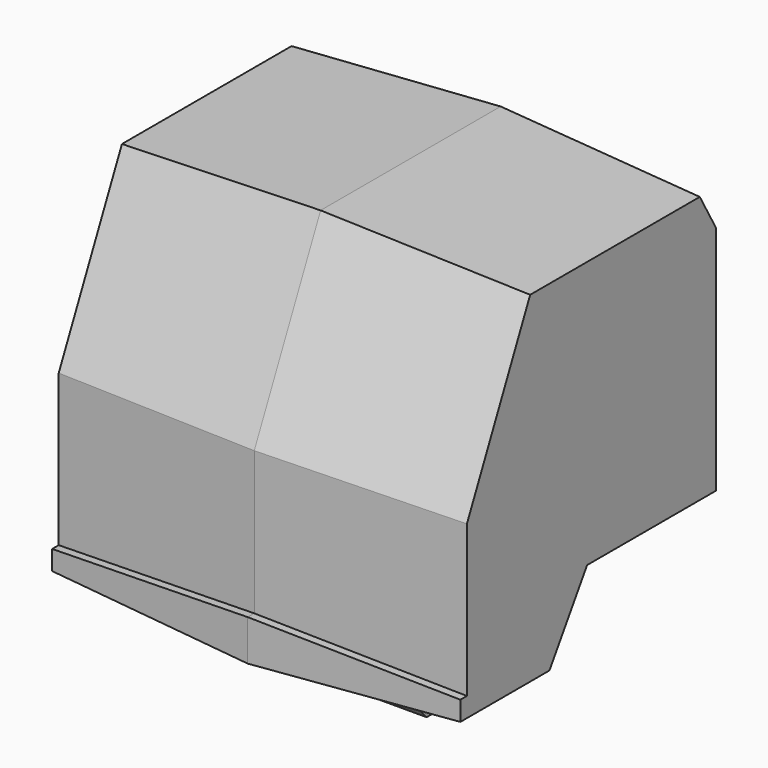
from build123d import *

# Parameters (mm, degrees)
F1_DEPTH = 997.5
F1_TAPER = 3
F3_DEPTH = 450


# Not quite as in the source:
# - a feature of the source that left no trace in its solid (it failed there, or was rolled back) is left out


with BuildPart() as f1:
    # F0 (on Right) → F1 (new body, symmetric)
    with BuildSketch(Plane.YZ):
        Polygon((-270, 660), (540, 660), (540, 1859), (420, 2069), (-679.7786450633, 2069), (-1085, 1200), (-1085, 500), (-1125, 500), (-1125, 300), (-500, 300), align=None)
    extrude(amount=F1_DEPTH, both=True, taper=F1_TAPER)

    # F2 (on Right) → F3 (join, symmetric)
    with BuildSketch(Plane.YZ):
        Polygon((540, 391.706943512), (540, 660), (540, 735.2597117424), (-594.5192575455, 735.2597117424), (-956.7571282387, 397.828578949), (-594.5192575455, 0), (0, 0), align=None)
    extrude(amount=F3_DEPTH, both=True)


solid = f1.part
